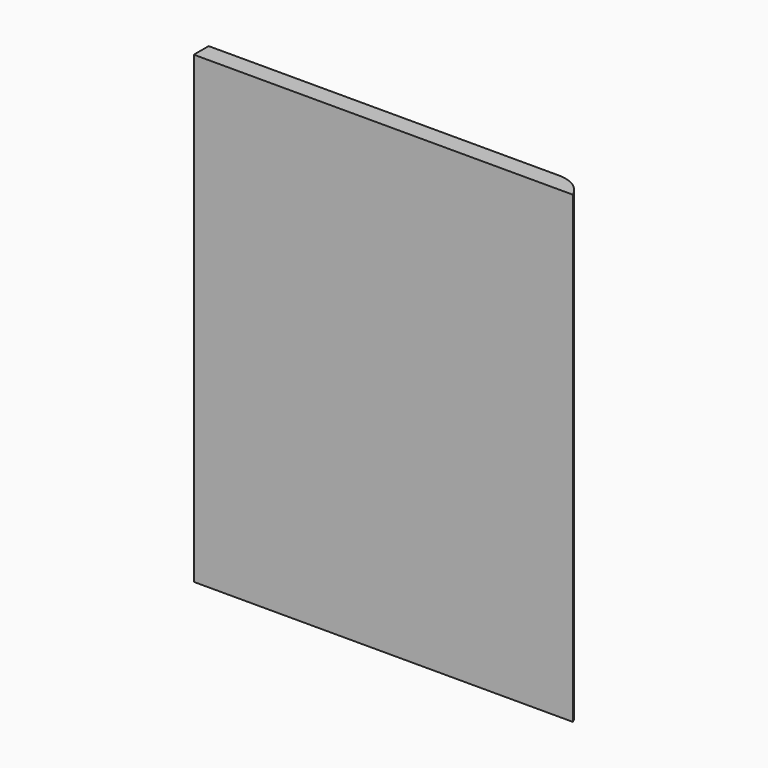
from build123d import *

# Parameters (mm, degrees)
F0_W        = 24.5
F0_H        = 30
F1_DEPTH    = 1.2
F2_T1_DEPTH = 39.1651513899


# Not quite as in the source:
# - a fillet or chamfer that OpenCascade refuses, or shapes differently, is made with other operations: its cross-section is extruded or revolved along the edge and cut away or added


with BuildPart() as f1:
    # F0 (on Front) → F1 (new body)
    with BuildSketch(Plane.XZ):
        Rectangle(F0_W, F0_H)
    extrude(amount=F1_DEPTH)

    # F2: fillet of radius 2 on 1 edges, made by hand

    # F2_s2 → F2_t1 (cut)
    with BuildSketch(Plane.XY.offset(-19.582575695)):
        with BuildLine():
            ThreePointArc((12.25, -1.2), (11.512414837, -0.3266799469), (10.416969722, 0))
            Line((10.416969722, 0), (12.25, 0))
            Line((12.25, 0), (12.25, -1.2))
        make_face()
    extrude(amount=F2_T1_DEPTH, mode=Mode.SUBTRACT)


solid = f1.part
